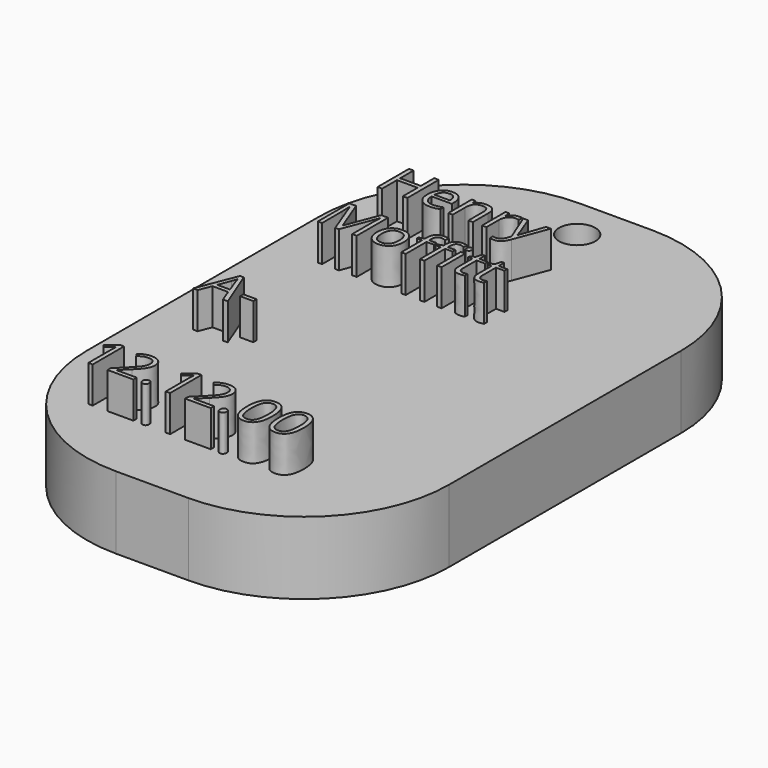
from build123d import *

# Parameters (mm, degrees)
F0_W         = 50
F0_H         = 80
F1_DEPTH     = 10
F2_R         = 20
F4_D         = 5
F5_TEXT_SIZE = 7.5743649336
F6_DEPTH     = 5


# Not quite as in the source:
# - Text() gives the source's letters only with a copy of the font that has no kerning and outlines rounded to 1/6400 em; it was checked with that copy


with BuildPart() as f1:
    # F0 (on Top) → F1 (new body)
    with BuildSketch(Plane.XY):
        with Locations((-45.167440176, 29.214329049)):
            Rectangle(F0_W, F0_H)
    extrude(amount=F1_DEPTH)

    # F2
    f2_edges = [f1.edges().sort_by_distance(p)[0] for p in [
        (-70.16744, -10.785671, 5),
        (-20.16744, -10.785671, 5),
        (-20.16744, 69.214329, 5),
        (-70.16744, 69.214329, 5),
    ]]
    fillet(f2_edges, radius=F2_R)

    # F4 (through all)
    with Locations(Plane.XY.offset(10)):
        with Locations((-45.8468981087, 63.3733719587)):
            Hole(F4_D / 2)

    # F5 (on face) → F6 (join)
    with BuildSketch(Plane.XY.offset(10)):
        with Locations((-64.3095757997, 51.1135645211)):
            Text('Henry', F5_TEXT_SIZE, font='Open Sans', text_align=(TextAlign.LEFT, TextAlign.BOTTOM))
        with Locations((-64.3095757997, 40.8124282114)):
            Text('Moffitt', F5_TEXT_SIZE, font='Open Sans', text_align=(TextAlign.LEFT, TextAlign.BOTTOM))
        with Locations((-64.3095757997, 20.2101555921)):
            Text('A-', F5_TEXT_SIZE, font='Open Sans', text_align=(TextAlign.LEFT, TextAlign.BOTTOM))
        with Locations((-64.3095757997, -0.3921170272)):
            Text('12.12.00', F5_TEXT_SIZE, font='Open Sans', text_align=(TextAlign.LEFT, TextAlign.BOTTOM))
    extrude(amount=F6_DEPTH)


solid = f1.part
